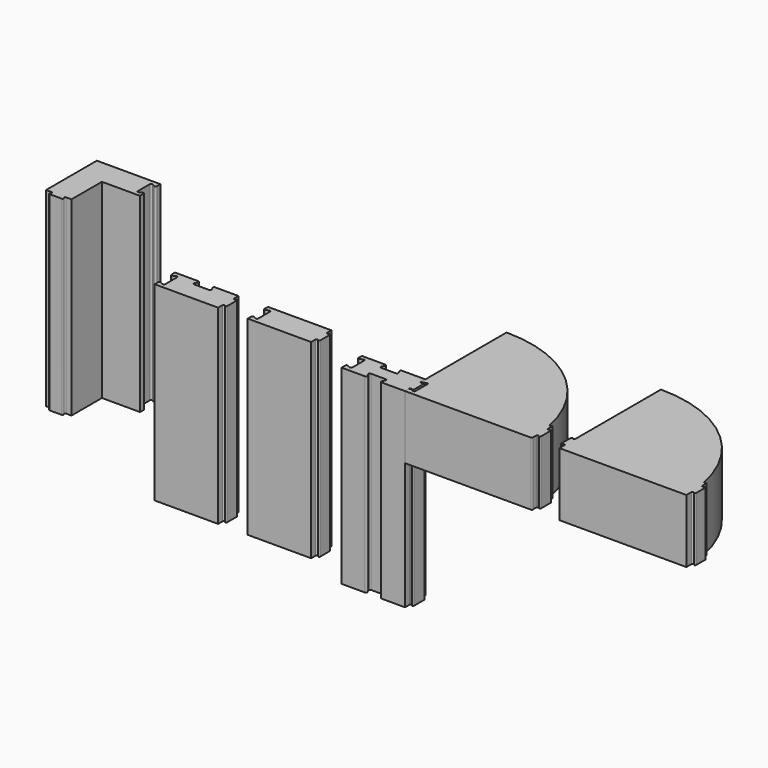
from build123d import *

# Parameters (mm, degrees)
F1_DEPTH  = 30
F3_DEPTH  = 10
F4_R      = 0.2
F5_R      = 0.16
F7_DEPTH  = 10
F8_R      = 0.16
F11_DEPTH = 30
F12_R     = 0.16
F13_R     = 0.2
F15_DEPTH = 30
F16_R     = 0.2
F17_R     = 0.16
F19_DEPTH = 30
F20_R     = 0.2
F21_R     = 0.16


# Not quite as in the source:
# - two fillets or chamfers of one size are made in one step


with BuildPart() as f1:
    # F0 (on Top) → F1 (new body)
    with BuildSketch(Plane.XY):
        with BuildLine():
            Line((1.3236067977, -2), (5, -2))
            Line((5, -2), (5, -1.0989058258))
            ThreePointArc((5, -1.0989058258), (5.0806182445, -0.9721233068), (5.229625816, -0.9913548466))
            Line((5.229625816, -0.9913548466), (5.370374184, -1.1086451534))
            ThreePointArc((5.370374184, -1.1086451534), (5.5193817555, -1.1278766932), (5.6, -1.0010941742))
            Line((5.6, -1.0010941742), (5.6, 0))
            Line((5.6, 0), (5.6, 1.0010941742))
            ThreePointArc((5.6, 1.0010941742), (5.5193817555, 1.1278766932), (5.370374184, 1.1086451534))
            Line((5.370374184, 1.1086451534), (5.229625816, 0.9913548466))
            ThreePointArc((5.229625816, 0.9913548466), (5.0806182445, 0.9721233068), (5, 1.0989058258))
            Line((5, 1.0989058258), (5, 2))
            Line((5, 2), (1.3236067977, 2))
            ThreePointArc((1.3236067977, 2), (1.1534766361, 1.9051462224), (1.1447213595, 1.7105572809))
            Line((1.1447213595, 1.7105572809), (1.3552786405, 1.2894427191))
            ThreePointArc((1.3552786405, 1.2894427191), (1.3465233639, 1.0948537776), (1.1763932023, 1))
            Line((1.1763932023, 1), (0, 1))
            Line((0, 1), (-1.1763932023, 1))
            ThreePointArc((-1.1763932023, 1), (-1.3465233639, 1.0948537776), (-1.3552786405, 1.2894427191))
            Line((-1.3552786405, 1.2894427191), (-1.1447213595, 1.7105572809))
            ThreePointArc((-1.1447213595, 1.7105572809), (-1.1534766361, 1.9051462224), (-1.3236067977, 2))
            Line((-1.3236067977, 2), (-5, 2))
            Line((-5, 2), (-5, 1.3335920057))
            ThreePointArc((-5, 1.3335920057), (-4.9028404642, 1.1620582221), (-4.7057616108, 1.1571858663))
            Line((-4.7057616108, 1.1571858663), (-4.2942383892, 1.3770267725))
            ThreePointArc((-4.2942383892, 1.3770267725), (-4.0971595358, 1.3721544167), (-4, 1.2006206331))
            Line((-4, 1.2006206331), (-4, 0.0342126388))
            Line((-4, 0.0342126388), (-4, -1.1321953555))
            ThreePointArc((-4, -1.1321953555), (-4.0971595358, -1.3037291391), (-4.2942383892, -1.3086014949))
            Line((-4.2942383892, -1.3086014949), (-4.7057616108, -1.0887605887))
            ThreePointArc((-4.7057616108, -1.0887605887), (-4.9028404642, -1.0936329445), (-5, -1.2651667281))
            Line((-5, -1.2651667281), (-5, -2))
            Line((-5, -2), (-1.3236067977, -2))
            ThreePointArc((-1.3236067977, -2), (-1.1534766361, -1.9051462224), (-1.1447213595, -1.7105572809))
            Line((-1.1447213595, -1.7105572809), (-1.3552786405, -1.2894427191))
            ThreePointArc((-1.3552786405, -1.2894427191), (-1.3465233639, -1.0948537776), (-1.1763932023, -1))
            Line((-1.1763932023, -1), (1.1763932023, -1))
            ThreePointArc((1.1763932023, -1), (1.3465233639, -1.0948537776), (1.3552786405, -1.2894427191))
            Line((1.3552786405, -1.2894427191), (1.1447213595, -1.7105572809))
            ThreePointArc((1.1447213595, -1.7105572809), (1.1534766361, -1.9051462224), (1.3236067977, -2))
        make_face()
    extrude(amount=F1_DEPTH)


with BuildPart() as f3:
    # F2 (on face) → F3 (new body)
    with BuildSketch(Plane.XY.offset(30)):
        with BuildLine():
            Line((5, -1.0989058258), (5, -2))
            Line((5, -2), (25, -2))
            Line((25, -2), (25, -0.8))
            Line((25, -0.8), (25.6, -1.3))
            Line((25.6, -1.3), (25.6, 0))
            Line((25.6, 0), (25.6, 1.3))
            Line((25.6, 1.3), (25, 0.8))
            Line((25, 0.8), (25, 2))
            Line((25, 2), (24.5959179423, 2))
            ThreePointArc((24.5959179423, 2), (17.6491106407, 13.4919333848), (5, 18))
            Line((5, 18), (5, 2))
            Line((5, 2), (5, 1.0989058258))
            ThreePointArc((5, 1.0989058258), (5.0073151868, 1.0542433095), (5.0284962908, 1.0142481454))
            Line((5.0284962908, 1.0142481454), (6, 1.5))
            Line((6, 1.5), (6, 0))
            Line((6, 0), (6, -1.5))
            Line((6, -1.5), (5.0284962908, -1.0142481454))
            ThreePointArc((5.0284962908, -1.0142481454), (5.0073151868, -1.0542433095), (5, -1.0989058258))
        make_face()
    extrude(amount=-F3_DEPTH)

    # F4
    f4_edges = [f3.edges().sort_by_distance(p)[0] for p in [
        (5.028496, 1.014248, 25),
        (6, 1.5, 25),
        (6, -1.5, 25),
        (5.028496, -1.014248, 25),
    ]]
    fillet(f4_edges, radius=F4_R)

    # F5
    f5_edges = [f3.edges().sort_by_distance(p)[0] for p in [
        (25, -2, 25),
        (25, -0.8, 25),
        (25.6, -1.3, 25),
        (25, 0.8, 25),
        (25.6, 1.3, 25),
    ]]
    fillet(f5_edges, radius=F5_R)


with BuildPart() as f7:
    # F6 (on face) → F7 (new body)
    with BuildSketch(Plane.XY.offset(30)):
        with BuildLine():
            Line((29.330952093, -0.5351407344), (29.330952093, -2))
            Line((29.330952093, -2), (39.330952093, -2))
            Line((39.330952093, -2), (49.330952093, -2))
            Line((49.330952093, -2), (49.330952093, -0.5351407344))
            Line((49.330952093, -0.5351407344), (49.930952093, -1.3))
            Line((49.930952093, -1.3), (49.930952093, 0))
            Line((49.930952093, 0), (49.930952093, 1.3))
            Line((49.930952093, 1.3), (49.330952093, 0.8))
            Line((49.330952093, 0.8), (49.330952093, 2))
            Line((49.330952093, 2), (48.9268700353, 2))
            ThreePointArc((48.9268700353, 2), (41.9800627337, 13.4919333848), (29.330952093, 18))
            Line((29.330952093, 18), (29.330952093, 0.8))
            Line((29.330952093, 0.8), (28.730952093, 1.3))
            Line((28.730952093, 1.3), (28.730952093, -1.3))
            Line((28.730952093, -1.3), (29.330952093, -0.5351407344))
        make_face()
    extrude(amount=-F7_DEPTH)

    # F8
    f8_edges = [f7.edges().sort_by_distance(p)[0] for p in [
        (29.330952, -0.535141, 25),
        (28.730952, -1.3, 25),
        (28.730952, 1.3, 25),
        (29.330952, 0.8, 25),
        (49.330952, 0.8, 25),
        (49.930952, 1.3, 25),
        (49.930952, -1.3, 25),
        (49.330952, -0.535141, 25),
    ]]
    fillet(f8_edges, radius=F8_R)


with BuildPart() as f11:
    # F10 (on face) → F11 (new body)
    with BuildSketch(Plane.XY.offset(30)):
        Polygon((-62.9702135921, 22.2567461804), (-62.9702135921, 12.2567461804), (-61.7702135921, 12.2567461804), (-62.2702135921, 11.6567461804), (-59.6702135921, 11.6567461804), (-60.1702135921, 12.2567461804), (-58.9702135921, 12.2567461804), (-58.9702135921, 18.2567461804), (-52.9702135921, 18.2567461804), (-52.9702135921, 19.2567461804), (-53.9702135921, 18.7567461804), (-53.9702135921, 21.7567461804), (-52.9702135921, 21.2567461804), (-52.9702135921, 22.2567461804), align=None)
    extrude(amount=-F11_DEPTH)

    # F12
    f12_edges = [f11.edges().sort_by_distance(p)[0] for p in [
        (-59.670214, 11.656746, 15),
        (-62.270214, 11.656746, 15),
        (-61.770214, 12.256746, 15),
        (-60.170214, 12.256746, 15),
    ]]
    fillet(f12_edges, radius=F12_R)

    # F13
    f13_edges = [f11.edges().sort_by_distance(p)[0] for p in [
        (-52.970214, 21.256746, 15),
        (-53.970214, 21.756746, 15),
        (-52.970214, 19.256746, 15),
        (-53.970214, 18.756746, 15),
    ]]
    fillet(f13_edges, radius=F13_R)


with BuildPart() as f15:
    # F14 (on face) → F15 (new body)
    with BuildSketch(Plane.XY.offset(30)):
        Polygon((-32.8436782062, 4.9894726099), (-36.8436782062, 4.9894726099), (-36.8436782062, 3.9894726099), (-35.8436782062, 4.4894726099), (-35.8436782062, 1.4894726099), (-36.8436782062, 1.9894726099), (-36.8436782062, 0.9894726099), (-26.8436782062, 0.9894726099), (-26.8436782062, 2.1894726099), (-26.2436782062, 1.6894726099), (-26.2436782062, 4.2894726099), (-26.8436782062, 3.7894726099), (-26.8436782062, 4.9894726099), (-30.8436782062, 4.9894726099), (-30.3436782062, 3.9894726099), (-33.3436782062, 3.9894726099), align=None)
    extrude(amount=-F15_DEPTH)

    # F16
    f16_edges = [f15.edges().sort_by_distance(p)[0] for p in [
        (-36.843678, 3.989473, 15),
        (-35.843678, 4.489473, 15),
        (-35.843678, 1.489473, 15),
        (-36.843678, 1.989473, 15),
        (-32.843678, 4.989473, 15),
        (-30.843678, 4.989473, 15),
        (-30.343678, 3.989473, 15),
        (-33.343678, 3.989473, 15),
    ]]
    fillet(f16_edges, radius=F16_R)

    # F17
    f17_edges = [f15.edges().sort_by_distance(p)[0] for p in [
        (-26.243678, 4.289473, 15),
        (-26.243678, 1.689473, 15),
        (-26.843678, 3.789473, 15),
        (-26.843678, 2.189473, 15),
    ]]
    fillet(f17_edges, radius=F17_R)


with BuildPart() as f19:
    # F18 (on face) → F19 (new body)
    with BuildSketch(Plane.XY.offset(30)):
        Polygon((-22.188315168, 1.9894726099), (-22.188315168, 0.9894726099), (-12.188315168, 0.9894726099), (-12.188315168, 2.1894726099), (-11.588315168, 1.6894726099), (-11.588315168, 4.2894726099), (-12.188315168, 3.7894726099), (-12.188315168, 4.9894726099), (-22.188315168, 4.9894726099), (-22.188315168, 3.9894726099), (-21.188315168, 4.4894726099), (-21.188315168, 1.4894726099), align=None)
    extrude(amount=-F19_DEPTH)

    # F20
    f20_edges = [f19.edges().sort_by_distance(p)[0] for p in [
        (-22.188315, 3.989473, 15),
        (-21.188315, 4.489473, 15),
        (-21.188315, 1.489473, 15),
        (-22.188315, 1.989473, 15),
    ]]
    fillet(f20_edges, radius=F20_R)

    # F21
    f21_edges = [f19.edges().sort_by_distance(p)[0] for p in [
        (-12.188315, 3.789473, 15),
        (-11.588315, 4.289473, 15),
        (-11.588315, 1.689473, 15),
        (-12.188315, 2.189473, 15),
    ]]
    fillet(f21_edges, radius=F21_R)


solid = Compound([f1.part, f3.part, f7.part, f11.part, f15.part, f19.part])
